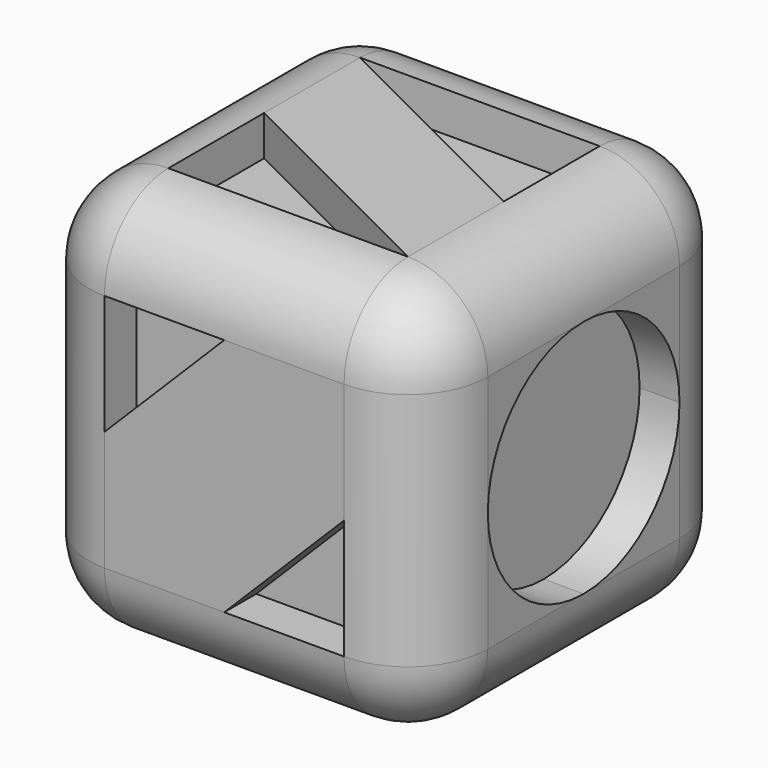
from build123d import *

# Parameters (mm, degrees)
F0_W      = 25.4
F0_H      = 25.4
F1_DEPTH  = 25.4
F2_R      = 5.08
F3_DEPTH  = 2.54
F4_DEPTH  = 2.54
F5_DEPTH  = 2.54
F6_DEPTH  = 2.54
F7_DEPTH  = 2.54
F8_DEPTH  = 2.54
F15_DEPTH = 2.54
F11_W     = 7.62
F11_H     = 7.62
F16_DEPTH = 2.54
F17_DEPTH = 2.54
F18_DEPTH = 2.54
F19_DEPTH = 2.54
F20_DEPTH = 2.54


with BuildPart() as f1:
    # F0 (on Front) → F1 (new body)
    with BuildSketch(Plane.XZ):
        with Locations((12.7, 12.7)):
            Rectangle(F0_W, F0_H)
    extrude(amount=F1_DEPTH)

    # F2
    f2_edges = [f1.edges().sort_by_distance(p)[0] for p in [
        (12.7, -25.4, 25.4),
        (12.7, -25.4, 0),
        (12.7, 0, 25.4),
        (12.7, 0, 0),
        (25.4, 0, 12.7),
        (0, 0, 12.7),
        (0, -12.7, 25.4),
        (0, -12.7, 0),
        (25.4, -12.7, 25.4),
        (25.4, -25.4, 12.7),
        (0, -25.4, 12.7),
        (25.4, -12.7, 0),
    ]]
    fillet(f2_edges, radius=F2_R)

    # F3 (cut): a face of the model
    f3_faces = [f1.faces().sort_by_distance(p)[0] for p in [
        (12.7, -25.4, 12.7),
    ]]
    extrude(f3_faces, amount=-F3_DEPTH, mode=Mode.SUBTRACT)

    # F4 (cut): a face of the model
    f4_faces = [f1.faces().sort_by_distance(p)[0] for p in [
        (0, -12.7, 12.7),
    ]]
    extrude(f4_faces, amount=-F4_DEPTH, mode=Mode.SUBTRACT)

    # F5 (cut): a face of the model
    f5_faces = [f1.faces().sort_by_distance(p)[0] for p in [
        (12.7, -12.7, 25.4),
    ]]
    extrude(f5_faces, amount=-F5_DEPTH, mode=Mode.SUBTRACT)

    # F6 (cut): a face of the model
    f6_faces = [f1.faces().sort_by_distance(p)[0] for p in [
        (25.4, -12.7, 12.7),
    ]]
    extrude(f6_faces, amount=-F6_DEPTH, mode=Mode.SUBTRACT)

    # F7 (cut): a face of the model
    f7_faces = [f1.faces().sort_by_distance(p)[0] for p in [
        (12.7, -12.7, 0),
    ]]
    extrude(f7_faces, amount=-F7_DEPTH, mode=Mode.SUBTRACT)

    # F8 (cut): a face of the model
    f8_faces = [f1.faces().sort_by_distance(p)[0] for p in [
        (12.7, 0, 12.7),
    ]]
    extrude(f8_faces, amount=-F8_DEPTH, mode=Mode.SUBTRACT)

    # F14 (on face) → F15 (join)
    with BuildSketch(Plane.XY.offset(22.86)):
        Polygon((20.32, -20.32), (20.32, -12.7), (5.08, -5.08), (5.08, -12.7), align=None)
    extrude(amount=F15_DEPTH)

    # F11 (on face) → F16 (join)
    with BuildSketch(Plane(origin=(0, -2.54, 0), x_dir=(-1, 0, 0), z_dir=(0, 1, 0))):
        with Locations((-12.7, 12.7)):
            Rectangle(F11_W, F11_H)
    extrude(amount=F16_DEPTH)

    # F9 (on face) → F17 (join)
    with BuildSketch(Plane.XZ.offset(22.86)):
        Polygon((12.7, 5.08), (5.08, 12.7), (5.08, 5.08), align=None)
        Polygon((12.7, 20.32), (5.08, 12.7), (12.7, 5.08), (20.32, 12.7), align=None)
        Polygon((20.32, 20.32), (12.7, 20.32), (20.32, 12.7), align=None)
    extrude(amount=F17_DEPTH)

    # F12 (on face) → F18 (join)
    with BuildSketch(Plane(origin=(2.54, 0, 0), x_dir=(0, -1, 0), z_dir=(-1, 0, 0))):
        Polygon((16.51, 20.32), (12.7, 20.32), (8.89, 20.32), (8.89, 16.51), (5.08, 16.51), (5.08, 12.7), (5.08, 8.89), (8.89, 8.89), (8.89, 5.08), (12.7, 5.08), (16.51, 5.08), (16.51, 8.89), (20.32, 8.89), (20.32, 12.7), (20.32, 16.51), (16.51, 16.51), align=None)
    extrude(amount=F18_DEPTH)

    # F13 (on face) → F19 (join)
    with BuildSketch(Plane(origin=(0, 0, 2.54), x_dir=(1, 0, 0), z_dir=(0, 0, -1))):
        Polygon((12.7, 8.89), (20.32, 5.08), (20.32, 20.32), (12.7, 16.51), (5.08, 12.7), align=None)
        Polygon((5.08, 5.08), (12.7, 8.89), (5.08, 12.7), align=None)
        Polygon((5.08, 20.32), (5.08, 12.7), (12.7, 16.51), align=None)
    extrude(amount=F19_DEPTH)

    # F10 (on face) → F20 (join)
    with BuildSketch(Plane.YZ.offset(22.86)):
        with BuildLine():
            Line((-5.08, 5.08), (-5.08, 12.7))
            ThreePointArc((-5.08, 12.7), (-7.3118463274, 7.3118463274), (-12.7, 5.08))
            Line((-12.7, 5.08), (-5.08, 5.08))
        make_face()
        with BuildLine():
            ThreePointArc((-12.7, 20.32), (-7.3118463274, 18.0881536726), (-5.08, 12.7))
            Line((-5.08, 12.7), (-5.08, 20.32))
            Line((-5.08, 20.32), (-12.7, 20.32))
        make_face()
        with BuildLine():
            ThreePointArc((-20.32, 12.7), (-18.0881536726, 18.0881536726), (-12.7, 20.32))
            Line((-12.7, 20.32), (-20.32, 20.32))
            Line((-20.32, 20.32), (-20.32, 12.7))
        make_face()
        with BuildLine():
            Line((-20.32, 5.08), (-12.7, 5.08))
            ThreePointArc((-12.7, 5.08), (-18.0881536726, 7.3118463274), (-20.32, 12.7))
            Line((-20.32, 12.7), (-20.32, 5.08))
        make_face()
    extrude(amount=F20_DEPTH)


solid = f1.part
